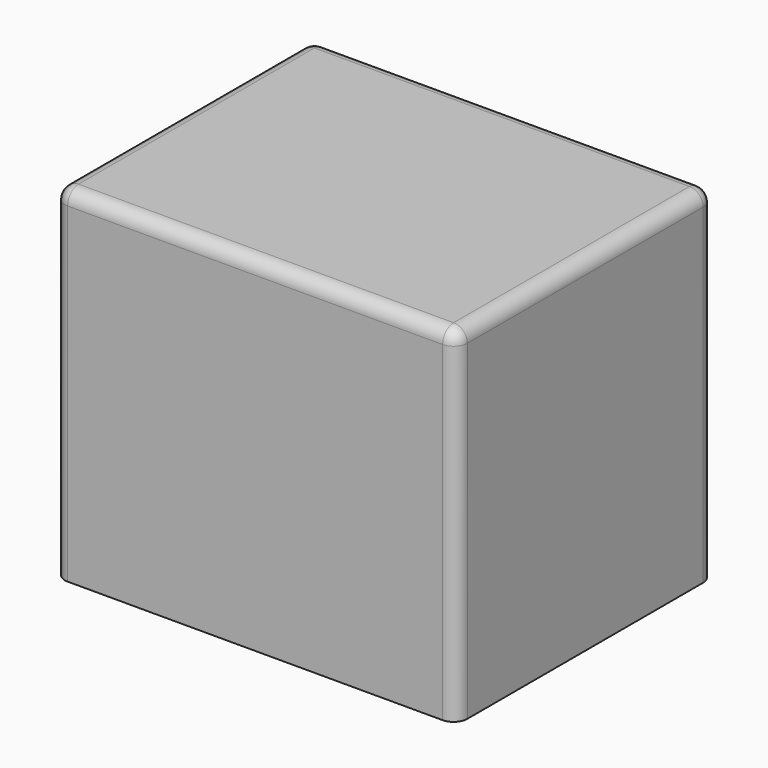
from build123d import *

# Parameters (mm, degrees)
F0_W        = 147.209584713
F0_H        = 117.8593859076
F1_DEPTH    = 126
F2_R        = 5
F3_T        = -2.5
F4_T1_DEPTH = 133.5
F4_S5_W     = 5
F4_S5_H     = 5
F4_T6_DEPTH = 5


# Not quite as in the source:
# - a fillet or chamfer that OpenCascade refuses, or shapes differently, is made with other operations: its cross-section is extruded or revolved along the edge and cut away or added


with BuildPart() as f1:
    # F0 (on Top) → F1 (new body)
    with BuildSketch(Plane.XY):
        Rectangle(F0_W, F0_H)
    extrude(amount=F1_DEPTH)

    # F2
    f2_edges = [f1.edges().sort_by_distance(p)[0] for p in [
        (-73.604792, -58.929693, 63),
        (73.604792, -58.929693, 63),
        (0, -58.929693, 126),
        (-73.604792, 0, 126),
        (0, 58.929693, 126),
        (73.604792, 0, 126),
        (-73.604792, 58.929693, 63),
    ]]
    fillet(f2_edges, radius=F2_R)

    # F3
    f3_openings = [f1.faces().sort_by_distance(p)[0] for p in [
        (0.022436, 0.017894, 0),
    ]]
    offset(amount=F3_T, openings=f3_openings)

    # F4: fillet of radius 5 on 1 edges, made by hand

    # F4_s2 → F4_t1 (cut)
    with BuildSketch(Plane.XY.offset(-12.5)):
        with BuildLine():
            ThreePointArc((73.6047923565, 53.9296929538), (72.1403262624, 57.4652268598), (68.6047923565, 58.9296929538))
            Line((68.6047923565, 58.9296929538), (73.6047923565, 58.9296929538))
            Line((73.6047923565, 58.9296929538), (73.6047923565, 53.9296929538))
        make_face()
    extrude(amount=F4_T1_DEPTH, mode=Mode.SUBTRACT)


with BuildPart() as f4_tool4:
    # F4_s5 → F4_t6 (new body)
    with BuildSketch(Plane.YZ.offset(68.6047923565)):
        with Locations((56.4296929538, 123.5)):
            Rectangle(F4_S5_W, F4_S5_H)
    extrude(amount=F4_T6_DEPTH)

    # F4_s7 → F4_t8 (revolve, cut)
    with BuildSketch(Plane(origin=(68.6047923565, 53.9296929538, 121), x_dir=(0, -0.7071067812, -0.7071067812), z_dir=(0, -0.7071067812, 0.7071067812))):
        with BuildLine():
            ThreePointArc((0, -5), (5, 0), (0, 5))
            Line((0, 5), (0, -5))
        make_face()
    revolve(axis=Axis((68.6047923565, 53.9296929538, 121), (1, 0, 0)), mode=Mode.SUBTRACT)


with BuildPart() as f1_1:
    add(f1.part)

    # F4_t3: cut F4_tool4
    add(f4_tool4.part, mode=Mode.SUBTRACT)


solid = f1_1.part
